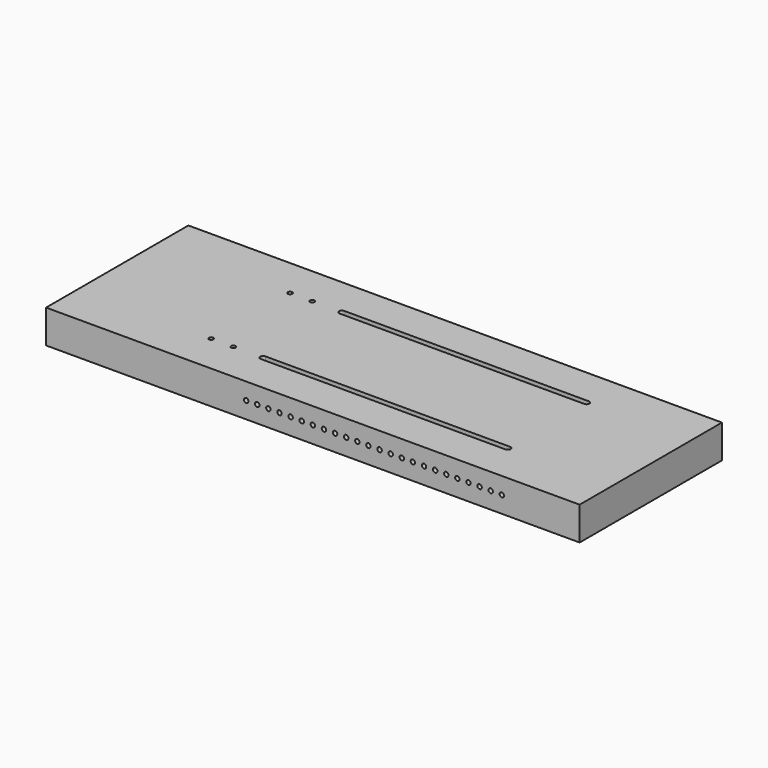
from build123d import *

# Parameters (mm, degrees)
F0_W      = 609.6
F0_H      = 38.1
F1_DEPTH  = 203.2
F3_D      = 5.1054
F5_D      = 5.1054
F5_DEPTH  = 25.4
F5_TIP    = 1.5338169022
F7_D      = 5.1054
F7_DEPTH  = 25.4
F7_TIP    = 1.5338169022
F8_R      = 5.08
F9_DEPTH  = 7.62
F12_DEPTH = 38.101


# Not quite as in the source:
# - the program builds the solid bodies; features that only make, move or delete a surface that nothing else refers to are left out


with BuildPart() as f1:
    # F0 (on Front) → F1 (new body)
    with BuildSketch(Plane.XZ):
        with Locations((304.8, 19.05)):
            Rectangle(F0_W, F0_H)
    extrude(amount=-F1_DEPTH)

    # F3 (through all)
    with Locations(Plane.XY.offset(38.1)):
        with Locations((152.4, 157.950154), (177.8, 157.950154), (152.4, 45.249846), (177.8, 45.249846)):
            Hole(F3_D / 2)

    # F5
    with Locations(Plane.XZ):
        with Locations((228.6, 19.05), (241.3, 19.05), (254, 19.05), (266.7, 19.05), (279.4, 19.05), (292.1, 19.05), (304.8, 19.05), (317.5, 19.05), (330.2, 19.05), (342.9, 19.05), (355.6, 19.05), (368.3, 19.05), (381, 19.05), (393.7, 19.05), (406.4, 19.05), (419.1, 19.05), (431.8, 19.05), (444.5, 19.05), (457.2, 19.05), (469.9, 19.05), (482.6, 19.05), (495.3, 19.05), (508, 19.05), (520.7, 19.05)):
            Hole(F5_D / 2, depth=F5_DEPTH)
            with Locations((0, 0, -(F5_DEPTH + F5_TIP / 2))):  # 118° drill point
                Cone(0, F5_D / 2, F5_TIP, mode=Mode.SUBTRACT)

    # F7
    with Locations(Plane(origin=(0, 203.2, 0), x_dir=(-1, 0, 0), z_dir=(0, 1, 0))):
        with Locations((-228.6, 19.05), (-241.3, 19.05), (-254, 19.05), (-266.7, 19.05), (-279.4, 19.05), (-292.1, 19.05), (-304.8, 19.05), (-317.5, 19.05), (-330.2, 19.05), (-342.9, 19.05), (-355.6, 19.05), (-368.3, 19.05), (-381, 19.05), (-393.7, 19.05), (-406.4, 19.05), (-419.1, 19.05), (-431.8, 19.05), (-444.5, 19.05), (-457.2, 19.05), (-469.9, 19.05), (-482.6, 19.05), (-495.3, 19.05), (-508, 19.05), (-520.7, 19.05)):
            Hole(F7_D / 2, depth=F7_DEPTH)
            with Locations((0, 0, -(F7_DEPTH + F7_TIP / 2))):  # 118° drill point
                Cone(0, F7_D / 2, F7_TIP, mode=Mode.SUBTRACT)

    # F8 (on face) → F9 (cut)
    with BuildSketch(Plane(origin=(0, 0, 0), x_dir=(1, 0, 0), z_dir=(0, 0, -1))):
        with Locations((177.8, -157.950154)):
            Circle(F8_R)
        with Locations((152.4, -157.950154)):
            Circle(F8_R)
        with Locations((177.8, -45.249846)):
            Circle(F8_R)
        with Locations((152.4, -45.249846)):
            Circle(F8_R)
    extrude(amount=-F9_DEPTH, mode=Mode.SUBTRACT)

    # F11 (on face) → F12 (cut, through all)
    with BuildSketch(Plane(origin=(0, 0, 0), x_dir=(1, 0, 0), z_dir=(0, 0, -1))):
        with BuildLine():
            ThreePointArc((211.7379009724, -154.5971), (208.4740009724, -157.861), (211.7379009724, -161.1249))
            Line((211.7379009724, -161.1249), (491.1379009724, -161.1249))
            ThreePointArc((491.1379009724, -161.1249), (494.4018009724, -157.861), (491.1379009724, -154.5971))
            Line((491.1379009724, -154.5971), (211.7379009724, -154.5971))
        make_face()
        with BuildLine():
            ThreePointArc((211.7379009724, -42.0751), (208.4740009724, -45.339), (211.7379009724, -48.6029))
            Line((211.7379009724, -48.6029), (491.1379009724, -48.6029))
            ThreePointArc((491.1379009724, -48.6029), (494.4018009724, -45.339), (491.1379009724, -42.0751))
            Line((491.1379009724, -42.0751), (211.7379009724, -42.0751))
        make_face()
    extrude(amount=-F12_DEPTH, mode=Mode.SUBTRACT)


solid = f1.part
